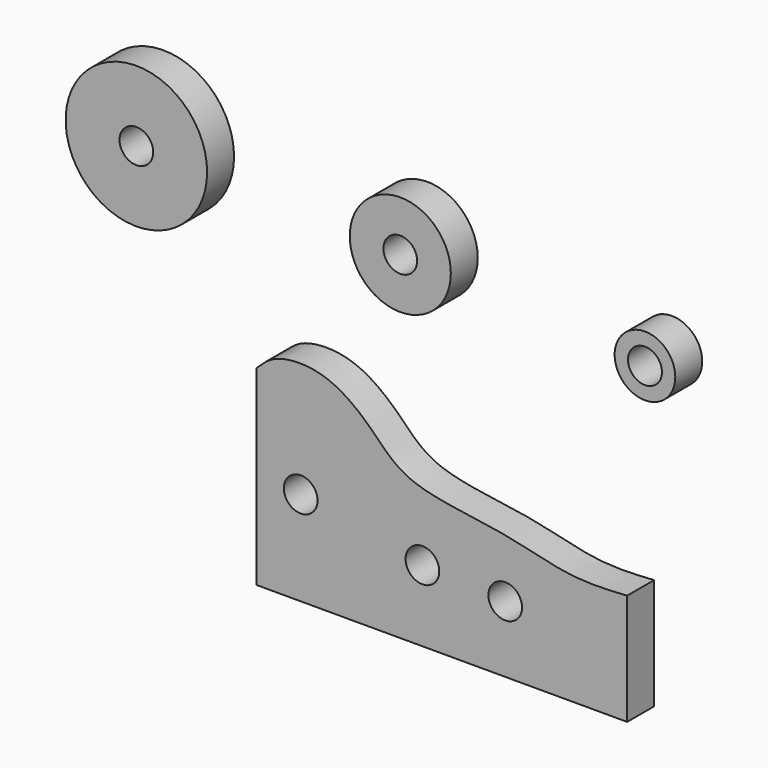
from build123d import *

# Parameters (mm, degrees)
F1_DEPTH = 6.35
F2_R     = 13.335
F2_R_2   = 3.175
F3_DEPTH = 6.35
F2_R_3   = 9.525
F4_DEPTH = 6.35
F2_R_4   = 5.715
F2_R_5   = 3.199782715
F7_D     = 6.35
F9_D     = 6.35
F11_D    = 6.35


with BuildPart() as f1:
    # F0 (on Front) → F1 (new body)
    with BuildSketch(Plane.XZ):
        with BuildLine():
            Line((-34.925, -20.955), (34.925, -20.955))
            Line((34.925, -20.955), (34.925, 0))
            add(Edge.make_bspline(
                [(-34.925, 15.0680310093), (-33.8749337765, 16.1178807955), (-31.3723698821, 18.6199288672), (-21.6066058687, 18.904040471), (-12.9641594898, 12.1368529586), (-6.9125027094, 4.5564810056), (11.3505046476, 3.3543035541), (23.9254899985, -0.6862175421), (31.4147522763, -0.2189909882), (34.925, 0)],
                knots=[0, 0, 0, 0, 0.095564903, 0.2277544697, 0.3722459873, 0.5069998522, 0.6921200679, 0.8556954222, 1, 1, 1, 1], degree=3))
            Line((-34.925, 15.0680310093), (-34.925, -20.955))
        make_face()
    extrude(amount=F1_DEPTH)

    # F7 (through all)
    with Locations(Plane.XZ.offset(6.35)):
        with Locations((-3.671587212, -7.4961567298)):
            Hole(F7_D / 2)

    # F9 (through all)
    with Locations(Plane.XZ.offset(6.35)):
        with Locations((-26.6190059483, -3.212638665)):
            Hole(F9_D / 2)

    # F11 (through all)
    with Locations(Plane.XZ.offset(6.35)):
        with Locations((11.9326571003, -8.4140533581)):
            Hole(F11_D / 2)


with BuildPart() as f3:
    # F2 (on Front) → F3 (new body)
    with BuildSketch(Plane.XZ):
        with Locations((-57.5947463512, 44.5191822946)):
            Circle(F2_R)
        with Locations((-57.5947463512, 44.5191822946)):
            Circle(F2_R_2, mode=Mode.SUBTRACT)
    extrude(amount=F3_DEPTH)


with BuildPart() as f3b:
    # F2 (on Front) → F3, piece 2 (new body)
    with BuildSketch(Plane.XZ):
        with Locations((-7.8441174701, 42.6720045507)):
            Circle(F2_R_3)
        with Locations((-7.8441174701, 42.6720045507)):
            Circle(F2_R_2, mode=Mode.SUBTRACT)
    extrude(amount=F3_DEPTH)


with BuildPart() as f4:
    # F2 (on Front) → F4 (new body)
    with BuildSketch(Plane.XZ):
        with Locations((-57.5947463512, 44.5191822946)):
            Circle(F2_R)
        with Locations((-57.5947463512, 44.5191822946)):
            Circle(F2_R_2, mode=Mode.SUBTRACT)
    extrude(amount=F4_DEPTH)


with BuildPart() as f4b:
    # F2 (on Front) → F4, piece 2 (new body)
    with BuildSketch(Plane.XZ):
        with Locations((-7.8441174701, 42.6720045507)):
            Circle(F2_R_3)
        with Locations((-7.8441174701, 42.6720045507)):
            Circle(F2_R_2, mode=Mode.SUBTRACT)
    extrude(amount=F4_DEPTH)


with BuildPart() as f4c:
    # F2 (on Front) → F4, piece 3 (new body)
    with BuildSketch(Plane.XZ):
        with Locations((38.2792986929, 39.2205901444)):
            Circle(F2_R_4)
        with Locations((38.2792986929, 39.2205901444)):
            Circle(F2_R_5, mode=Mode.SUBTRACT)
    extrude(amount=F4_DEPTH)


solid = Compound([f1.part, f3.part, f3b.part, f4.part, f4b.part, f4c.part])
